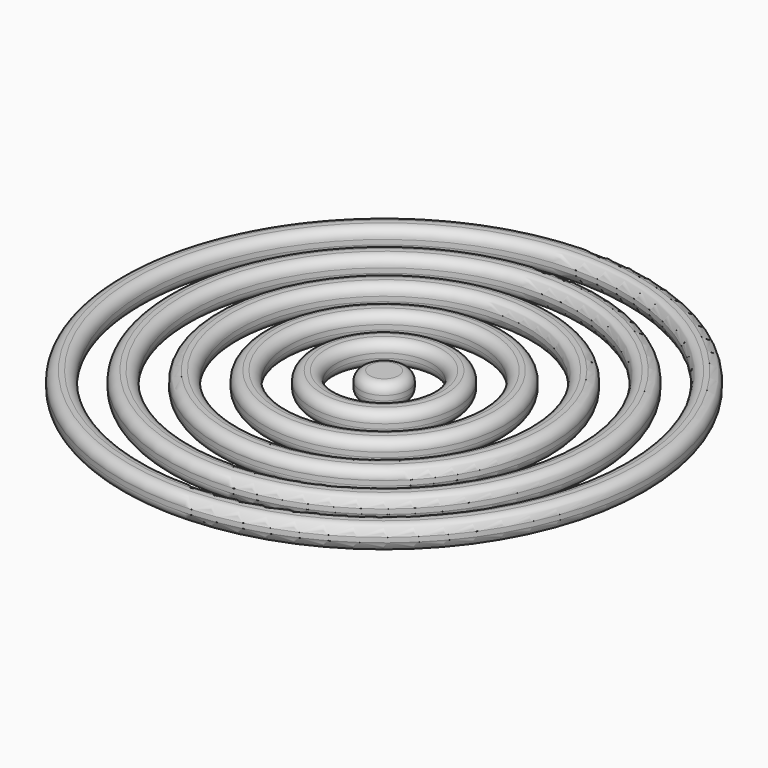
from build123d import *

# Parameters (mm, degrees)
F0_R     = 139.7
F0_R_2   = 127
F1_DEPTH = 12.7
F0_R_3   = 114.3
F0_R_4   = 101.6
F0_R_5   = 88.9
F0_R_6   = 76.2
F0_R_7   = 63.5
F0_R_8   = 50.8
F0_R_9   = 38.1
F0_R_10  = 25.4
F0_R_11  = 12.7
F2_R     = 5.08
F3_R     = 5.08
F4_R     = 5.08
F5_R     = 5.08
F6_R     = 5.08
F6_2_R   = 5.08


# Not quite as in the source:
# - a feature names something its author has since deleted; it is built from what else it names


with BuildPart() as f1:
    # F0 (on Top) → F1 (new body)
    with BuildSketch(Plane.XY):
        Circle(F0_R)
        Circle(F0_R_2, mode=Mode.SUBTRACT)
    extrude(amount=F1_DEPTH)

    # F6
    f6_edges = [f1.edges().sort_by_distance(p)[0] for p in [
        (-139.7, 0, 12.7),
        (-127, 0, 12.7),
        (-139.7, 0, 0),
        (-127, 0, 0),
        (127, 0, 6.35),
        (139.7, 0, 6.35),
    ]]
    fillet(f6_edges, radius=F6_R)


with BuildPart() as f1b:
    # F0 (on Top) → F1, piece 2 (new body)
    with BuildSketch(Plane.XY):
        Circle(F0_R_3)
        Circle(F0_R_4, mode=Mode.SUBTRACT)
    extrude(amount=F1_DEPTH)

    # F6#2
    f6_2_edges = [f1b.edges().sort_by_distance(p)[0] for p in [
        (101.6, 0, 6.35),
        (-101.6, 0, 0),
        (-101.6, 0, 12.7),
        (-114.3, 0, 0),
        (-114.3, 0, 12.7),
        (114.3, 0, 6.35),
    ]]
    fillet(f6_2_edges, radius=F6_2_R)


with BuildPart() as f1c:
    # F0 (on Top) → F1, piece 3 (new body)
    with BuildSketch(Plane.XY):
        Circle(F0_R_5)
        Circle(F0_R_6, mode=Mode.SUBTRACT)
    extrude(amount=F1_DEPTH)

    # F5
    f5_edges = [f1c.edges().sort_by_distance(p)[0] for p in [
        (76.2, 0, 6.35),
        (-76.2, 0, 0),
        (-76.2, 0, 12.7),
        (-88.9, 0, 12.7),
        (-88.9, 0, 0),
        (88.9, 0, 6.35),
    ]]
    fillet(f5_edges, radius=F5_R)


with BuildPart() as f1d:
    # F0 (on Top) → F1, piece 4 (new body)
    with BuildSketch(Plane.XY):
        Circle(F0_R_7)
        Circle(F0_R_8, mode=Mode.SUBTRACT)
    extrude(amount=F1_DEPTH)

    # F4
    f4_edges = [f1d.edges().sort_by_distance(p)[0] for p in [
        (-63.5, 0, 12.7),
        (-50.8, 0, 12.7),
        (50.8, 0, 6.35),
        (-50.8, 0, 0),
        (-63.5, 0, 0),
        (63.5, 0, 6.35),
    ]]
    fillet(f4_edges, radius=F4_R)


with BuildPart() as f1e:
    # F0 (on Top) → F1, piece 5 (new body)
    with BuildSketch(Plane.XY):
        Circle(F0_R_9)
        Circle(F0_R_10, mode=Mode.SUBTRACT)
    extrude(amount=F1_DEPTH)

    # F3
    f3_edges = [f1e.edges().sort_by_distance(p)[0] for p in [
        (38.1, 0, 6.35),
        (-38.1, 0, 0),
        (-38.1, 0, 12.7),
        (-25.4, 0, 12.7),
        (-25.4, 0, 0),
        (25.4, 0, 6.35),
    ]]
    fillet(f3_edges, radius=F3_R)


with BuildPart() as f1f:
    # F0 (on Top) → F1, piece 6 (new body)
    with BuildSketch(Plane.XY):
        Circle(F0_R_11)
    extrude(amount=F1_DEPTH)

    # F2
    f2_edges = [f1f.edges().sort_by_distance(p)[0] for p in [
        (-12.7, 0, 0),
        (12.7, 0, 6.35),
        (-12.7, 0, 12.7),
    ]]
    fillet(f2_edges, radius=F2_R)


solid = Compound([f1.part, f1b.part, f1c.part, f1d.part, f1e.part, f1f.part])
